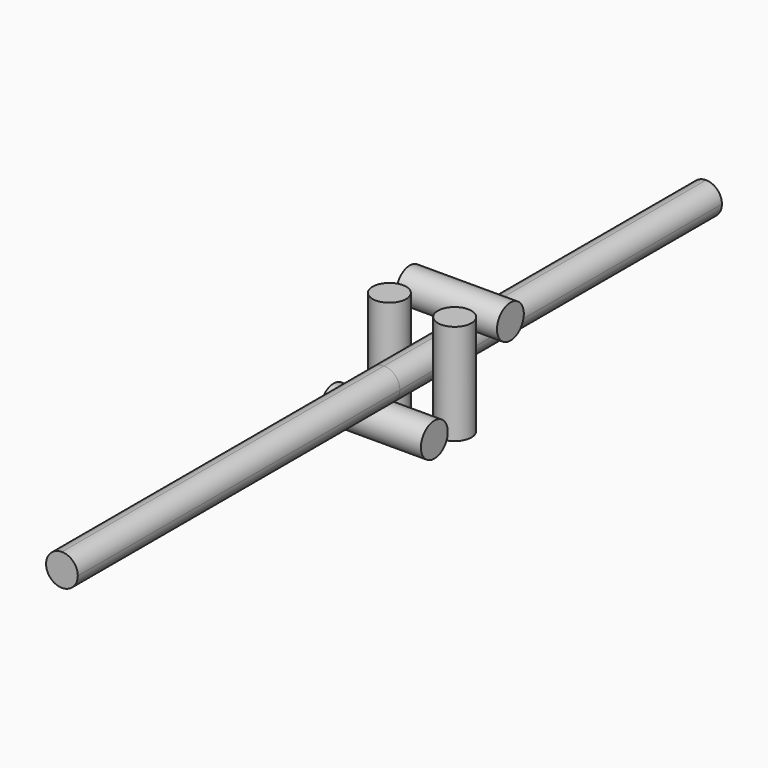
from build123d import *

# Parameters (mm, degrees)
F1_DEPTH        = 38.1
F2_COPIES_COUNT = 2
F2_COPIES_PITCH = 10.914698
F3_R            = 1.5875
F4_DEPTH        = 4.7625


# Not quite as in the source:
# - a feature of the source that left no trace in its solid (it failed there, or was rolled back) is left out
# - a length typed as a fraction of an inch, garbled in the dataset ("3 / 203.2 mm" for 3/8 in), is restored
# - a pattern or mirror of a feature is missing from the dataset's text; its kind, count and spacing are read off the source's solid


with BuildPart() as f1:
    # F0 (on Front) → F1 (new body, symmetric)
    with BuildSketch(Plane.XZ):
        with BuildLine():
            ThreePointArc((0, -1.5), (1.0606601718, -1.0606601718), (1.5, 0))
            ThreePointArc((1.5, 0), (1.0606601718, 1.0606601718), (0, 1.5))
            ThreePointArc((0, 1.5), (-1.5, 0), (0, -1.5))
        make_face()
    extrude(amount=F1_DEPTH, both=True)


with BuildPart() as f2:
    # F0 (on Front) → F2 (revolve)
    with BuildSketch(Plane.XZ):
        Polygon((4.7625, -1.5), (0, -1.5), (-4.7625, -1.5), (-4.7625, -3.0875), (4.7625, -3.0875), align=None)
    revolve(axis=Axis((0, 0, -3.0875), (1, 0, 0)))


with BuildPart() as f2_copies_1:
    # F2_copies: instance of F2
    add(f2.part.moved(Location(Vector(0, 0.8245762073, 0.5657508978) * (1 * F2_COPIES_PITCH))))


with BuildPart() as f4:
    # F3 (on Top) → F4 (new body, symmetric)
    with BuildSketch(Plane.XY):
        with Locations((3.0875, 4.5)):
            Circle(F3_R)
    extrude(amount=F4_DEPTH, both=True)


with BuildPart() as f4b:
    # F3 (on Top) → F4, piece 2 (new body, symmetric)
    with BuildSketch(Plane.XY):
        with Locations((-3.0875, 4.5)):
            Circle(F3_R)
    extrude(amount=F4_DEPTH, both=True)


solid = Compound([f1.part, f2.part, f2_copies_1.part, f4.part, f4b.part])
